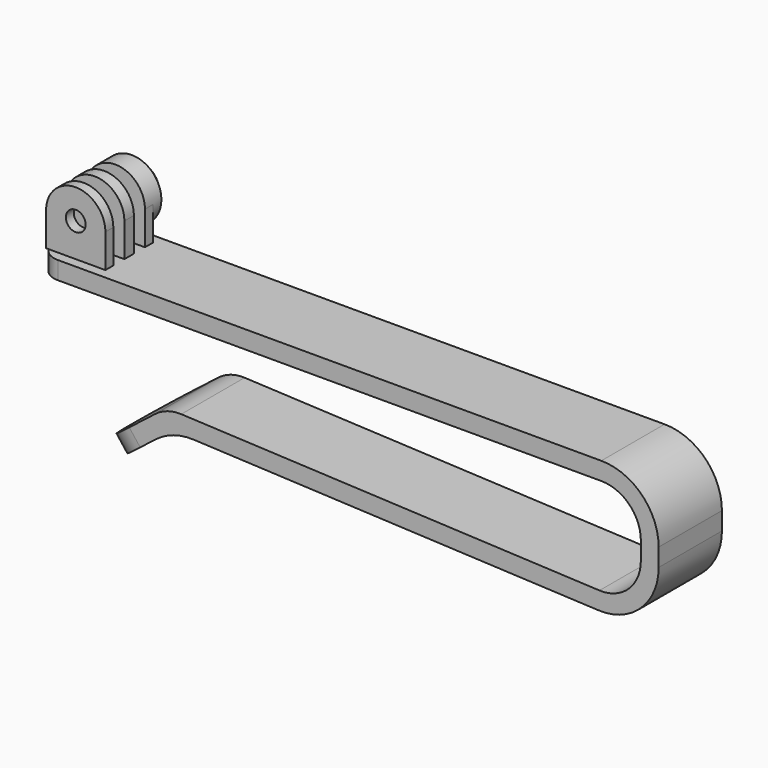
from build123d import *

# Parameters (mm, degrees)
F0_R     = 2.5
F1_DEPTH = 1.5
F2_START = 5
F2_DEPTH = 2.5
F3_START = -5
F3_DEPTH = 2.5
F4_START = -7.5
F4_DEPTH = 4.7
F5_SIZE  = 2
F7_DEPTH = 10
F8_R     = 10
F9_R     = 14.5
F10_R    = 9.99999
F11_R    = 5


# Not quite as in the source:
# - a fillet or chamfer is up to 0.001 mm smaller than in the source, because OpenCascade refuses the exact size


with BuildPart() as f1:
    # F0 (on Front) → F1 (new body, symmetric)
    with BuildSketch(Plane.XZ):
        with BuildLine():
            Line((7.5, -8.5), (7.5, 0))
            ThreePointArc((7.5, 0), (0, -7.5), (-7.5, 0))
            Line((-7.5, 0), (-7.5, -8.5))
            Line((-7.5, -8.5), (7.5, -8.5))
        make_face()
        with BuildLine():
            ThreePointArc((-7.5, 0), (0, -7.5), (7.5, 0))
            ThreePointArc((7.5, 0), (0, 7.5), (-7.5, 0))
        make_face()
        Polygon((2.1975, 3.8061816496), (4.395, 0), (2.1975, -3.8061816496), (-2.1975, -3.8061816496), (-4.395, 0), (-2.1975, 3.8061816496), align=None, mode=Mode.SUBTRACT)
        Polygon((2.1975, -3.8061816496), (4.395, 0), (2.1975, 3.8061816496), (-2.1975, 3.8061816496), (-4.395, 0), (-2.1975, -3.8061816496), align=None)
        Circle(F0_R, mode=Mode.SUBTRACT)
    extrude(amount=F1_DEPTH, both=True)


with BuildPart() as f2:
    # F0 (on Front) → F2 (new body)
    with BuildSketch(Plane.XZ.offset(F2_START)):
        with BuildLine():
            Line((7.5, -8.5), (7.5, 0))
            ThreePointArc((7.5, 0), (0, -7.5), (-7.5, 0))
            Line((-7.5, 0), (-7.5, -8.5))
            Line((-7.5, -8.5), (7.5, -8.5))
        make_face()
        with BuildLine():
            ThreePointArc((-7.5, 0), (0, -7.5), (7.5, 0))
            ThreePointArc((7.5, 0), (0, 7.5), (-7.5, 0))
        make_face()
        Polygon((2.1975, 3.8061816496), (4.395, 0), (2.1975, -3.8061816496), (-2.1975, -3.8061816496), (-4.395, 0), (-2.1975, 3.8061816496), align=None, mode=Mode.SUBTRACT)
        Polygon((2.1975, -3.8061816496), (4.395, 0), (2.1975, 3.8061816496), (-2.1975, 3.8061816496), (-4.395, 0), (-2.1975, -3.8061816496), align=None)
        Circle(F0_R, mode=Mode.SUBTRACT)
    extrude(amount=F2_DEPTH)


with BuildPart() as f3:
    # F0 (on Front) → F3 (new body)
    with BuildSketch(Plane.XZ.offset(F3_START)):
        with BuildLine():
            ThreePointArc((-7.5, 0), (0, -7.5), (7.5, 0))
            ThreePointArc((7.5, 0), (0, 7.5), (-7.5, 0))
        make_face()
        Polygon((2.1975, 3.8061816496), (4.395, 0), (2.1975, -3.8061816496), (-2.1975, -3.8061816496), (-4.395, 0), (-2.1975, 3.8061816496), align=None, mode=Mode.SUBTRACT)
        with BuildLine():
            Line((7.5, -8.5), (7.5, 0))
            ThreePointArc((7.5, 0), (0, -7.5), (-7.5, 0))
            Line((-7.5, 0), (-7.5, -8.5))
            Line((-7.5, -8.5), (7.5, -8.5))
        make_face()
        Polygon((2.1975, -3.8061816496), (4.395, 0), (2.1975, 3.8061816496), (-2.1975, 3.8061816496), (-4.395, 0), (-2.1975, -3.8061816496), align=None)
        Circle(F0_R, mode=Mode.SUBTRACT)
    extrude(amount=-F3_DEPTH)

    # F0 (on Front) → F4 (join)
    with BuildSketch(Plane.XZ.offset(F4_START)):
        with BuildLine():
            ThreePointArc((-7.5, 0), (0, -7.5), (7.5, 0))
            ThreePointArc((7.5, 0), (0, 7.5), (-7.5, 0))
        make_face()
        Polygon((2.1975, 3.8061816496), (4.395, 0), (2.1975, -3.8061816496), (-2.1975, -3.8061816496), (-4.395, 0), (-2.1975, 3.8061816496), align=None, mode=Mode.SUBTRACT)
    extrude(amount=-F4_DEPTH)

    # F5
    f5_edges = [f3.edges().sort_by_distance(p)[0] for p in [
        (-7.5, 12.2, 0),
    ]]
    chamfer(f5_edges, length=F5_SIZE)


with BuildPart() as f7:
    # F6 (on Front) → F7 (new body, symmetric)
    with BuildSketch(Plane.XZ):
        Polygon((149.4, -8.5), (-7.5, -8.5), (-7.5, -13), (144.9, -13), (144.9, -38), (25, -32.5), (7.6514315894, -46.028753605), (10.418676645, -49.5773244162), (26.4554967217, -37.0714978667), (149.4, -42.7111539804), align=None)
    extrude(amount=F7_DEPTH, both=True)

    # F8
    f8_edges = [f7.edges().sort_by_distance(p)[0] for p in [
        (25, 0, -32.5),
        (144.9, 0, -38),
        (144.9, 0, -13),
    ]]
    fillet(f8_edges, radius=F8_R)

    # F9
    f9_edges = [f7.edges().sort_by_distance(p)[0] for p in [
        (149.4, 0, -42.711154),
        (149.4, 0, -8.5),
        (26.455497, 0, -37.071498),
    ]]
    fillet(f9_edges, radius=F9_R)

    # F10 (radius 10 in the source; OpenCascade refuses exactly that, so slightly less here)
    f10_edges = [f7.edges().sort_by_distance(p)[0] for p in [
        (9.035054, 10, -47.803039),
        (9.035054, -10, -47.803039),
    ]]
    fillet(f10_edges, radius=F10_R)

    # F11
    f11_edges = [f7.edges().sort_by_distance(p)[0] for p in [
        (-7.5, -10, -10.75),
        (-7.5, 10, -10.75),
    ]]
    fillet(f11_edges, radius=F11_R)


solid = Compound([f1.part, f2.part, f3.part, f7.part])
